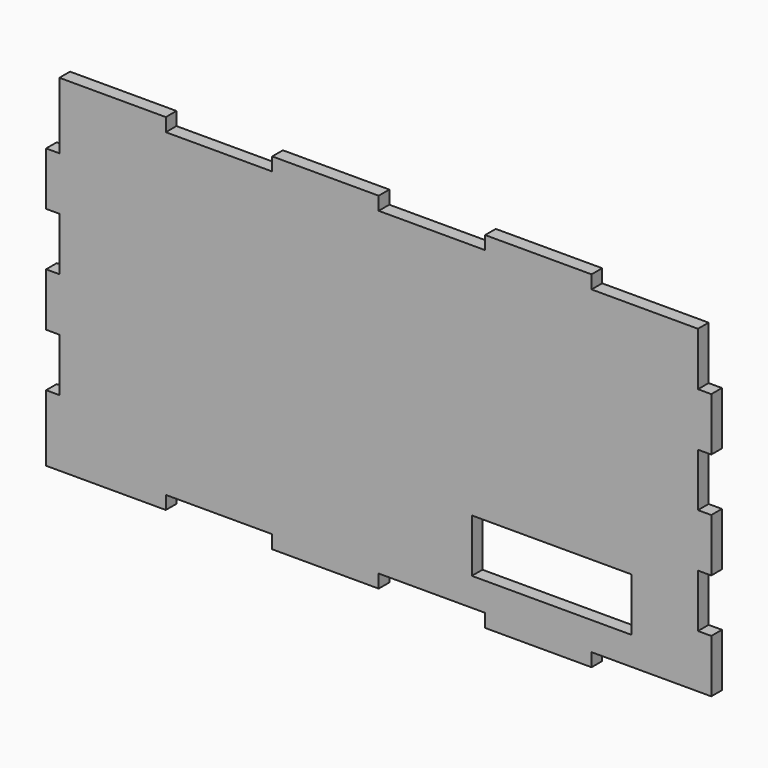
from build123d import *

# Parameters (mm, degrees)
F1_DEPTH = 3.175
F2_W     = 38.1
F2_H     = 12.7
F3_DEPTH = 25.4


# Not quite as in the source:
# - a length typed as a fraction of an inch, garbled in the dataset ("3 / 203.2 mm" for 3/8 in), is restored


with BuildPart() as f1:
    # F0 (on Front) → F1 (new body)
    with BuildSketch(Plane.XZ):
        Polygon((15.2796131081, -5.7429333596), (15.2796131081, 6.9570666404), (-10.1203868919, 6.9570666404), (-10.1203868919, 10.1320666404), (-35.5203868919, 10.1320666404), (-35.5203868919, 6.9570666404), (-60.9203868919, 6.9570666404), (-60.9203868919, 10.1320666404), (-86.3203868919, 10.1320666404), (-86.3203868919, 6.9570666404), (-111.7203868919, 6.9570666404), (-111.7203868919, 10.1320666404), (-137.1203868919, 10.1320666404), (-137.1203868919, 6.9570666404), (-137.1203868919, -5.7429333596), (-140.2953868919, -5.7429333596), (-140.2953868919, -18.4429333596), (-137.1203868919, -18.4429333596), (-137.1203868919, -31.1429333596), (-140.2953868919, -31.1429333596), (-140.2953868919, -43.8429333596), (-137.1203868919, -43.8429333596), (-137.1203868919, -56.5429333596), (-140.2953868919, -56.5429333596), (-140.2953868919, -69.2429333596), (-140.2953868919, -72.4179333596), (-137.1203868919, -72.4179333596), (-111.7203868919, -72.4179333596), (-111.7203868919, -69.2429333596), (-86.3203868919, -69.2429333596), (-86.3203868919, -72.4179333596), (-60.9203868919, -72.4179333596), (-60.9203868919, -69.2429333596), (-35.5203868919, -69.2429333596), (-35.5203868919, -72.4179333596), (-10.1203868919, -72.4179333596), (-10.1203868919, -69.2429333596), (15.2796131081, -69.2429333596), (18.4546131081, -69.2429333596), (18.4546131081, -56.5429333596), (15.2796131081, -56.5429333596), (15.2796131081, -43.8429333596), (18.4546131081, -43.8429333596), (18.4546131081, -31.1429333596), (15.2796131081, -31.1429333596), (15.2796131081, -18.4429333596), (18.4546131081, -18.4429333596), (18.4546131081, -5.7429333596), align=None)
    extrude(amount=F1_DEPTH)

    # F2 (on face) → F3 (cut)
    with BuildSketch(Plane.XZ.offset(3.175)):
        with Locations((-19.6453868919, -56.1550986022)):
            Rectangle(F2_W, F2_H)
    extrude(amount=-F3_DEPTH, mode=Mode.SUBTRACT)


solid = f1.part
